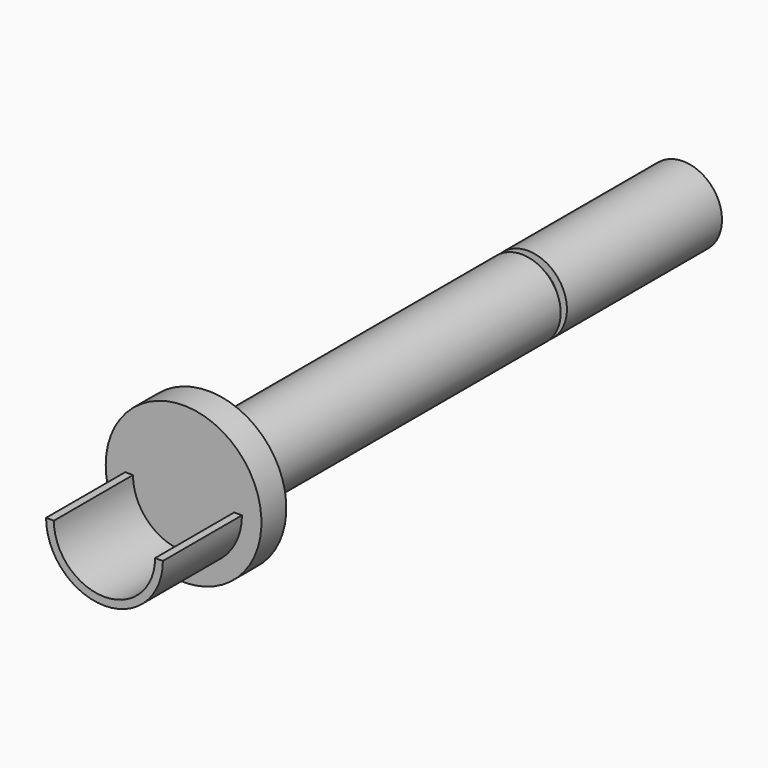
from build123d import *

# Parameters (mm, degrees)
F1_DEPTH = 25.4
F2_R     = 20
F3_DEPTH = 8
F4_R     = 10
F5_DEPTH = 152.4
F7_R     = 12.7
F7_R_2   = 8
F8_DEPTH = 1


with BuildPart() as f1:
    # F0 (on Front) → F1 (new body)
    with BuildSketch(Plane.XZ):
        with BuildLine():
            Line((-13, 0), (-15, 0))
            ThreePointArc((-15, 0), (0, -15), (15, 0))
            Line((15, 0), (13, 0))
            ThreePointArc((13, 0), (0, -13), (-13, 0))
        make_face()
    extrude(amount=-F1_DEPTH)


with BuildPart() as f3:
    # F2 (on face) → F3 (new body)
    with BuildSketch(Plane(origin=(0, 25.4, 0), x_dir=(-1, 0, 0), z_dir=(0, 1, 0))):
        Circle(F2_R)
        with BuildLine():
            Line((-15, 0), (-13, 0))
            ThreePointArc((-13, 0), (0, -13), (13, 0))
            Line((13, 0), (15, 0))
            ThreePointArc((15, 0), (0, -15), (-15, 0))
        make_face(mode=Mode.SUBTRACT)
        with BuildLine():
            ThreePointArc((13, 0), (0, -13), (-13, 0))
            Line((-13, 0), (-15, 0))
            ThreePointArc((-15, 0), (0, -15), (15, 0))
            Line((15, 0), (13, 0))
        make_face()
    extrude(amount=F3_DEPTH)

    # F4 (on face) → F5 (join)
    with BuildSketch(Plane(origin=(0, 33.4, 0), x_dir=(-1, 0, 0), z_dir=(0, 1, 0))):
        Circle(F4_R)
    extrude(amount=F5_DEPTH)

    # F7 (on offset) → F8 (cut, symmetric)
    with BuildSketch(Plane(origin=(0, 135, 0), x_dir=(-1, 0, 0), z_dir=(0, 1, 0))):
        Circle(F7_R)
        Circle(F7_R_2, mode=Mode.SUBTRACT)
    extrude(amount=F8_DEPTH, both=True, mode=Mode.SUBTRACT)


solid = Compound([f1.part, f3.part])
